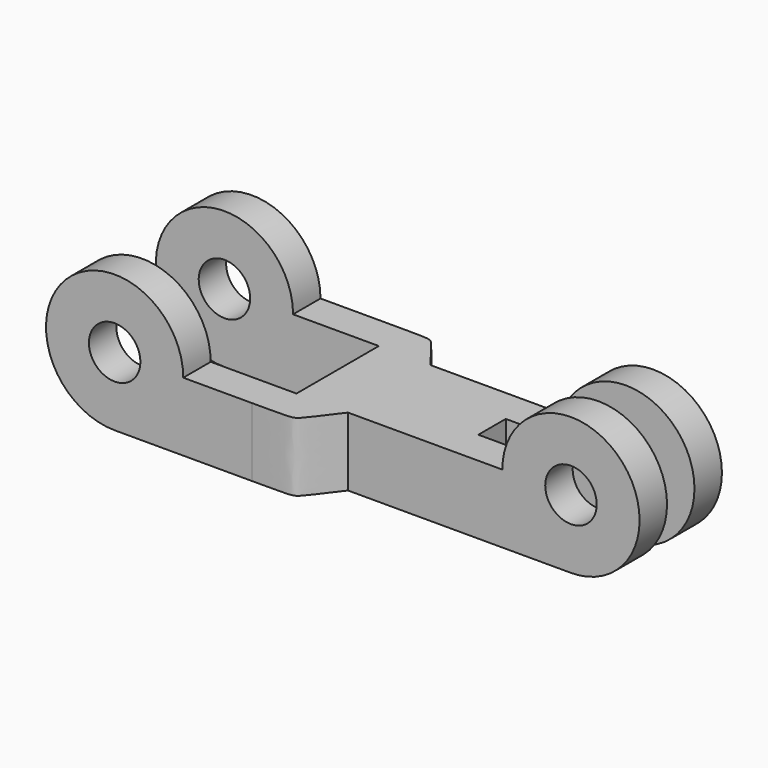
from build123d import *

# Parameters (mm, degrees)
F0_W        = 3
F0_H        = 4
F1_DEPTH    = 5
F0_W_2      = 6
F2_DEPTH    = 3
F3_DEPTH    = 3
F4_DEPTH    = 1
F5_T1_DEPTH = 24


# Not quite as in the source:
# - a fillet or chamfer that OpenCascade refuses, or shapes differently, is made with other operations: its cross-section is extruded or revolved along the edge and cut away or added


with BuildPart() as f1:
    # F0 (on Front) → F1 (new body, symmetric)
    with BuildSketch(Plane.XZ):
        with BuildLine():
            Line((-11, 2), (-8.5, 2))
            ThreePointArc((-8.5, 2), (-15.3284271247, 4.8284271247), (-12.5, -2))
            Line((-12.5, -2), (-12.5, 0.5))
            ThreePointArc((-12.5, 0.5), (-13.5606601718, 3.0606601718), (-11, 2))
        make_face()
        with BuildLine():
            ThreePointArc((-12.5, -2), (-9.6715728753, -0.8284271247), (-8.5, 2))
            Line((-8.5, 2), (-11, 2))
            ThreePointArc((-11, 2), (-11.4393398282, 0.9393398282), (-12.5, 0.5))
            Line((-12.5, 0.5), (-12.5, -2))
        make_face()
        with BuildLine():
            Line((-3.5, -2), (-3.5, 2))
            Line((-3.5, 2), (-8.5, 2))
            ThreePointArc((-8.5, 2), (-9.6715728753, -0.8284271247), (-12.5, -2))
            Line((-12.5, -2), (-3.5, -2))
        make_face()
        with Locations((-2, 0)):
            Rectangle(F0_W, F0_H)
    extrude(amount=F1_DEPTH, both=True)

    # F0 (on Front) → F2 (join, symmetric)
    with BuildSketch(Plane.XZ):
        with Locations((2.5, 0)):
            Rectangle(F0_W_2, F0_H)
        with BuildLine():
            Line((8.5, 2), (5.5, 2))
            Line((5.5, 2), (5.5, -2))
            Line((5.5, -2), (12.5, -2))
            ThreePointArc((12.5, -2), (9.6715728753, -0.8284271247), (8.5, 2))
        make_face()
        with BuildLine():
            Line((11, 2), (8.5, 2))
            ThreePointArc((8.5, 2), (9.6715728753, -0.8284271247), (12.5, -2))
            Line((12.5, -2), (12.5, 0.5))
            ThreePointArc((12.5, 0.5), (11.4393398282, 0.9393398282), (11, 2))
        make_face()
        with BuildLine():
            ThreePointArc((16.5, 2), (12.5, 6), (8.5, 2))
            Line((8.5, 2), (11, 2))
            ThreePointArc((11, 2), (12.5, 3.5), (14, 2))
            ThreePointArc((14, 2), (13.5606601718, 0.9393398282), (12.5, 0.5))
            Line((12.5, 0.5), (12.5, -2))
            ThreePointArc((12.5, -2), (15.3284271247, -0.8284271247), (16.5, 2))
        make_face()
    extrude(amount=F2_DEPTH, both=True)

    # F0 (on Front) → F3 (cut, symmetric)
    with BuildSketch(Plane.XZ):
        with BuildLine():
            Line((-3.5, -2), (-3.5, 2))
            Line((-3.5, 2), (-8.5, 2))
            ThreePointArc((-8.5, 2), (-9.6715728753, -0.8284271247), (-12.5, -2))
            Line((-12.5, -2), (-3.5, -2))
        make_face()
        with BuildLine():
            ThreePointArc((-12.5, -2), (-9.6715728753, -0.8284271247), (-8.5, 2))
            Line((-8.5, 2), (-11, 2))
            ThreePointArc((-11, 2), (-11.4393398282, 0.9393398282), (-12.5, 0.5))
            Line((-12.5, 0.5), (-12.5, -2))
        make_face()
        with BuildLine():
            Line((-11, 2), (-8.5, 2))
            ThreePointArc((-8.5, 2), (-15.3284271247, 4.8284271247), (-12.5, -2))
            Line((-12.5, -2), (-12.5, 0.5))
            ThreePointArc((-12.5, 0.5), (-13.5606601718, 3.0606601718), (-11, 2))
        make_face()
    extrude(amount=F3_DEPTH, both=True, mode=Mode.SUBTRACT)

    # F0 (on Front) → F4 (cut, symmetric)
    with BuildSketch(Plane.XZ):
        with BuildLine():
            Line((8.5, 2), (5.5, 2))
            Line((5.5, 2), (5.5, -2))
            Line((5.5, -2), (12.5, -2))
            ThreePointArc((12.5, -2), (9.6715728753, -0.8284271247), (8.5, 2))
        make_face()
        with BuildLine():
            Line((11, 2), (8.5, 2))
            ThreePointArc((8.5, 2), (9.6715728753, -0.8284271247), (12.5, -2))
            Line((12.5, -2), (12.5, 0.5))
            ThreePointArc((12.5, 0.5), (11.4393398282, 0.9393398282), (11, 2))
        make_face()
        with BuildLine():
            ThreePointArc((16.5, 2), (12.5, 6), (8.5, 2))
            Line((8.5, 2), (11, 2))
            ThreePointArc((11, 2), (12.5, 3.5), (14, 2))
            ThreePointArc((14, 2), (13.5606601718, 0.9393398282), (12.5, 0.5))
            Line((12.5, 0.5), (12.5, -2))
            ThreePointArc((12.5, -2), (15.3284271247, -0.8284271247), (16.5, 2))
        make_face()
    extrude(amount=F4_DEPTH, both=True, mode=Mode.SUBTRACT)

    # F5: fillet of radius 5 on 2 edges, made by hand

    # F5_s2 → F5_t1 (cut)
    with BuildSketch(Plane.XY.offset(-12)):
        with BuildLine():
            add(Edge.make_bspline(
                [(-4.5, -5), (-2, -5), (-0.5, -3)],
                knots=[0, 0, 0, 1, 1, 1], degree=2, weights=[1, 9, 1]))
            Line((-0.5, -3), (-0.5, -5))
            Line((-0.5, -5), (-4.5, -5))
        make_face()
        with BuildLine():
            add(Edge.make_bspline(
                [(-4.5, 5), (-2, 5), (-0.5, 3)],
                knots=[0, 0, 0, 1, 1, 1], degree=2, weights=[1, 9, 1]))
            Line((-0.5, 3), (-0.5, 5))
            Line((-0.5, 5), (-4.5, 5))
        make_face()
    extrude(amount=F5_T1_DEPTH, mode=Mode.SUBTRACT)


solid = f1.part
